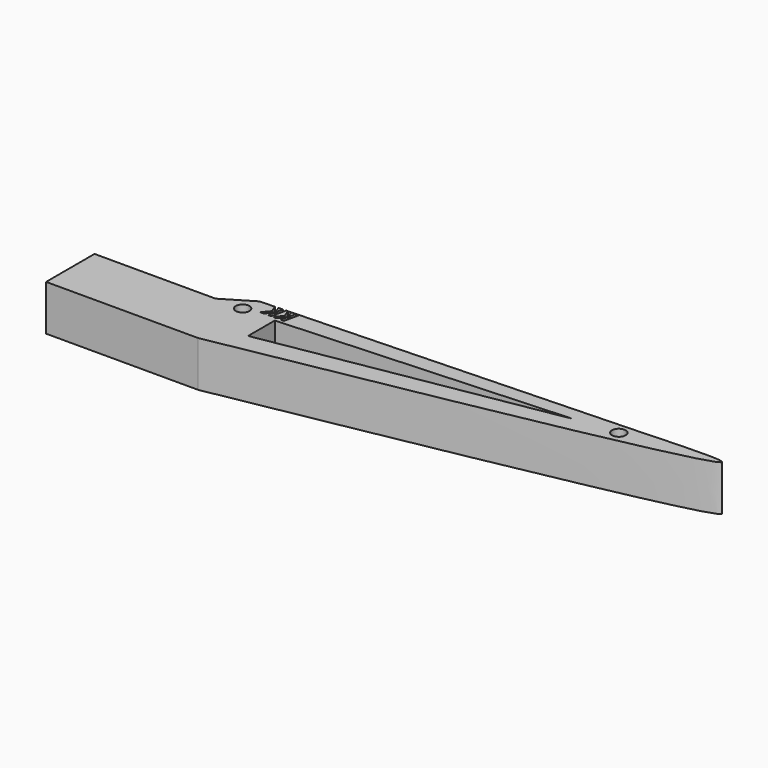
from build123d import *

# Parameters (mm, degrees)
F0_W         = 200
F0_H         = 50
F1_DEPTH     = 15
F2_R         = 5
F3_DEPTH     = 50
F4_R         = 2.25
F5_DEPTH     = 15.001
F6_DEPTH     = 15.001
F7_TEXT_SIZE = 6.831978
F8_DEPTH     = 5
F9_ANGLE     = -90


# Not quite as in the source:
# - a feature names something its author has since deleted; it is built from what else it names
# - Text() gives the source's letters only with a copy of the font that has no kerning and outlines rounded to 1/6400 em; it was checked with that copy


with BuildPart() as f1:
    # F0 (on Front) → F1 (new body)
    with BuildSketch(Plane.XZ):
        with Locations((15.800271, -7.299187)):
            Rectangle(F0_W, F0_H)
    extrude(amount=F1_DEPTH)

    # F2 (on face) → F3 (cut)
    with BuildSketch(Plane(origin=(-84.199729, 0, 0), x_dir=(0, -1, 0), z_dir=(-1, 0, 0))):
        with Locations((7.5, 5.559316)):
            Circle(F2_R)
    extrude(amount=-F3_DEPTH, mode=Mode.SUBTRACT)

    # F4 (on face) → F5 (cut, through all)
    with BuildSketch(Plane.XZ.offset(15)):
        with Locations((-35.561115, -2.25)):
            Circle(F4_R)
        with BuildLine():
            Line((-34.6525, -8.046538), (-44.395942, -2.203094))
            Line((-44.395942, -2.203094), (-84.199729, -2.203094))
            Line((-84.199729, -2.203094), (-84.199729, -7.299187))
            Line((-84.199729, -7.299187), (-84.199729, -32.299187))
            Line((-84.199729, -32.299187), (115.800271, -32.299187))
            Line((115.800271, -32.299187), (115.800271, 17.700813))
            Line((115.800271, 17.700813), (-34.183491, 17.700813))
            add(Edge.make_bspline(
                [(87.540562, -12.448189), (100.621768, -13.065235), (145.060332, -15.161422), (39.971062, 4.105453), (-34.183491, 17.700813)],
                knots=[0, 0, 0, 0, 0.294366, 1, 1, 1, 1], degree=3))
            Line((87.540562, -12.448189), (-34.6525, -8.046538))
        make_face()
        Polygon((69.061235, -7.299187), (-24.930276, 8.779588), (-24.930276, -2.203094), align=None)
        with Locations((83.01618, -8.642419)):
            Circle(F4_R)
    extrude(amount=-F5_DEPTH, mode=Mode.SUBTRACT)

    # F4 (on face) → F6 (cut, through all)
    with BuildSketch(Plane.XZ.offset(15)):
        with BuildLine():
            Line((-34.6525, -8.046538), (-44.395942, -2.203094))
            Line((-44.395942, -2.203094), (-84.199729, -2.203094))
            Line((-84.199729, -2.203094), (-84.199729, -7.299187))
            Line((-84.199729, -7.299187), (-84.199729, -32.299187))
            Line((-84.199729, -32.299187), (115.800271, -32.299187))
            Line((115.800271, -32.299187), (115.800271, 17.700813))
            Line((115.800271, 17.700813), (-34.183491, 17.700813))
            add(Edge.make_bspline(
                [(87.540562, -12.448189), (100.621768, -13.065235), (145.060332, -15.161422), (39.971062, 4.105453), (-34.183491, 17.700813)],
                knots=[0, 0, 0, 0, 0.294366, 1, 1, 1, 1], degree=3))
            Line((87.540562, -12.448189), (-34.6525, -8.046538))
        make_face()
    extrude(amount=-F6_DEPTH, mode=Mode.SUBTRACT)

    # F7 (on face) → F8 (cut)
    with BuildSketch(Plane(origin=(0, 0, 0), x_dir=(-1, 0, 0), z_dir=(0, 1, 0))):
        with Locations((21.74977, -8.348884)):
            Text('KK', F7_TEXT_SIZE, font='Open Sans', font_style=FontStyle.BOLDITALIC, text_align=(TextAlign.LEFT, TextAlign.BOTTOM))
    extrude(amount=-F8_DEPTH, mode=Mode.SUBTRACT)


with BuildPart() as f1_1:
    # F9: moved
    add(f1.part.rotate(Axis((-64.297836, -15, -2.203094), (-1, 0, 0)), F9_ANGLE))


solid = f1_1.part
